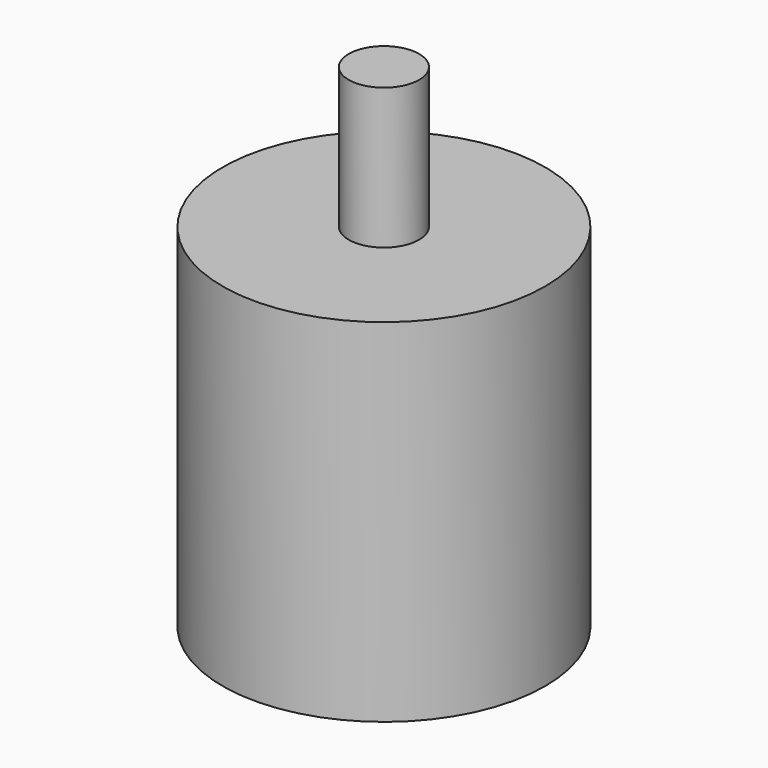
from build123d import *

# Parameters (mm, degrees)
F0_R     = 4.03124
F1_DEPTH = 4
F2_R     = 13.75
F3_DEPTH = 30
F4_R     = 3
F5_DEPTH = 12


# Not quite as in the source:
# - a feature names something its author has since deleted; it is built from what else it names


with BuildPart() as f1:
    # F0 (on Top) → F1 (new body)
    with BuildSketch(Plane.XY):
        Circle(F0_R)
    extrude(amount=F1_DEPTH)

    # F2 (on face) → F3 (join)
    with BuildSketch(Plane.XY.offset(4)):
        Circle(F2_R)
    extrude(amount=F3_DEPTH)

    # F4 (on face) → F5 (join)
    with BuildSketch(Plane.XY.offset(34)):
        Circle(F4_R)
    extrude(amount=F5_DEPTH)


solid = f1.part
